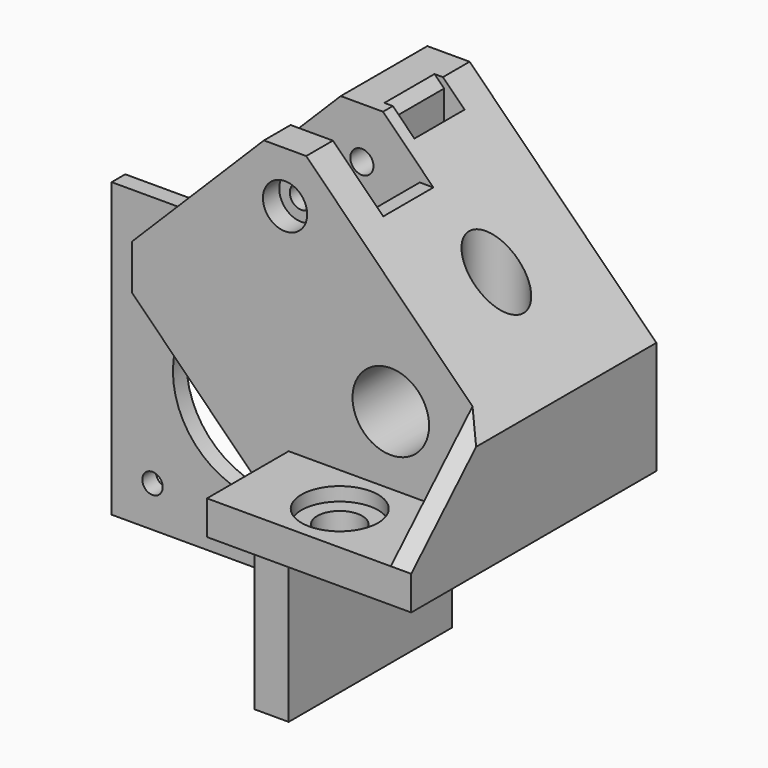
from build123d import *

# Parameters (mm, degrees)
F5_DEPTH        = 30
F7_DEPTH        = 27.5
F9_DEPTH        = 9.2
F11_DEPTH       = 9.2
F13_D           = 6.6
F13_CBORE_D     = 11.25
F13_CBORE_DEPTH = 27
F15_R           = 4
F16_DEPTH       = 39.001
F18_D           = 6.6
F18_CBORE_D     = 11.25
F18_CBORE_DEPTH = 2
F20_DEPTH       = 15
F22_D           = 6.6
F22_CBORE_D     = 11.25
F22_CBORE_DEPTH = 2
F24_DEPTH       = 3.001
F25_R           = 1.5
F25_R_2         = 12.5
F26_DEPTH       = 45.001
F28_D           = 3.4
F28_DEPTH       = 20
F28_CBORE_D     = 6.5
F28_CBORE_DEPTH = 3
F28_TIP         = 1.0214630523
F30_D           = 3.4
F30_DEPTH       = 20
F30_CBORE_D     = 6.5
F30_CBORE_DEPTH = 3
F30_TIP         = 1.0214630523
F31_SIZE        = 5


# Not quite as in the source:
# - a feature of the source that left no trace in its solid (it failed there, or was rolled back) is left out


with BuildPart() as f5:
    # F4 (on Front) → F5 (new body)
    with BuildSketch(Plane.XZ):
        Polygon((35, 46.5766017178), (7.5766017178, 74), (1.3633982822, 74), (-18.03, 54.6066017178), (-18.03, 43), (-43, 43), (-43, 0), (5, 0), (5, 30), (35, 30), align=None)
    extrude(amount=F5_DEPTH)

    # F6 (on face) → F7 (cut)
    with BuildSketch(Plane.XZ.offset(30)):
        Polygon((-43, 43), (-43, 0), (0, 0), (0, 30), (-18.03, 48.03), (-18.03, 43), align=None)
    extrude(amount=-F7_DEPTH, mode=Mode.SUBTRACT)

    # F8 (on offset) → F9 (cut)
    with BuildSketch(Plane.XZ.offset(14.1)):
        with BuildLine():
            Line((-18.03, 48.03), (-2.7734474577, 32.7734474577))
            Line((-2.7734474577, 32.7734474577), (9.5961081783, 47.0624990203))
            ThreePointArc((9.5961081783, 47.0624990203), (11.1595399436, 50.3961633531), (10.75, 54.0553864678))
            Line((10.75, 54.0553864678), (10.75, 70.8266017178))
            Line((10.75, 70.8266017178), (7.5766017178, 74))
            Line((7.5766017178, 74), (6.3357864376, 74))
            Line((6.3357864376, 74), (7.75, 72.5857864376))
            Line((7.75, 72.5857864376), (7.75, 61.4142135624))
            Line((7.75, 61.4142135624), (6.3357864376, 60))
            Line((6.3357864376, 60), (1.5055339059, 60))
            Line((1.5055339059, 60), (-5.5655339059, 67.0710678119))
            Line((-5.5655339059, 67.0710678119), (-18.03, 54.6066017178))
            Line((-18.03, 54.6066017178), (-18.03, 48.03))
        make_face()
    extrude(amount=-F9_DEPTH, mode=Mode.SUBTRACT)

    # F10 (on offset) → F11 (cut)
    with BuildSketch(Plane.XZ.offset(15.9)):
        with BuildLine():
            Line((1.3633982822, 74), (-16.6157864376, 56.0208152802))
            Line((-16.6157864376, 56.0208152802), (5.2500150699, 58.035865284))
            ThreePointArc((5.2500150699, 58.035865284), (10.7501324864, 60.7720041941), (12.97, 66.5))
            Line((12.97, 66.5), (12.97, 66.6066017178))
            Line((12.97, 66.6066017178), (14.97, 66.6066017178))
            Line((14.97, 66.6066017178), (7.5766017178, 74))
            Line((7.5766017178, 74), (1.3633982822, 74))
        make_face()
    extrude(amount=F11_DEPTH, mode=Mode.SUBTRACT)

    # F13 (through all)
    with Locations(Plane.XZ.offset(30)):
        with Locations((20, 45)):
            CounterBoreHole(F13_D / 2, F13_CBORE_D / 2, F13_CBORE_DEPTH)

    # F15 (on offset) → F16 (cut, through all)
    with BuildSketch(Plane(origin=(0, 0, 35), x_dir=(1, 0, 0), z_dir=(0, 0, -1))):
        with Locations((23.5, 15)):
            Circle(F15_R)
    extrude(amount=-F16_DEPTH, mode=Mode.SUBTRACT)

    # F18 (through all)
    with Locations(Plane(origin=(0, 0, 0), x_dir=(0, -1, 0), z_dir=(-1, 0, 0))):
        with Locations((16.25, 15)):
            CounterBoreHole(F18_D / 2, F18_CBORE_D / 2, F18_CBORE_DEPTH)

    # F19 (on face) → F20 (join)
    with BuildSketch(Plane.XZ.offset(30)):
        Polygon((5, 30), (35, 30), (35, 35), (35, 46.5766017178), (32, 49.5766017178), (32, 35), (5, 35), align=None)
    extrude(amount=F20_DEPTH)

    # F22 (through all)
    with Locations(Plane.XY.offset(35)):
        with Locations((18.5, -37.5)):
            CounterBoreHole(F22_D / 2, F22_CBORE_D / 2, F22_CBORE_DEPTH)

    # F23 (on face) → F24 (cut, through all)
    with BuildSketch(Plane(origin=(32, 0, 0), x_dir=(0, -1, 0), z_dir=(-1, 0, 0))):
        Polygon((45, 49.5766017178), (30, 49.5766017178), (45, 35), align=None)
    extrude(amount=-F24_DEPTH, mode=Mode.SUBTRACT)

    # F25 (on face) → F26 (cut, through all)
    with BuildSketch(Plane(origin=(0, 0, 0), x_dir=(-1, 0, 0), z_dir=(0, 1, 0))):
        with Locations((37, 37)):
            Circle(F25_R)
        with Locations((37, 6)):
            Circle(F25_R)
        with Locations((6, 6)):
            Circle(F25_R)
        with Locations((21.5, 21.5)):
            Circle(F25_R_2)
    extrude(amount=-F26_DEPTH, mode=Mode.SUBTRACT)

    # F28
    with Locations(Plane.XZ.offset(30)):
        with Locations((4.47, 66.5)):
            CounterBoreHole(F28_D / 2, F28_CBORE_D / 2, F28_CBORE_DEPTH, depth=F28_DEPTH)
            with Locations((0, 0, -(F28_DEPTH + F28_TIP / 2))):  # 118° drill point
                Cone(0, F28_D / 2, F28_TIP, mode=Mode.SUBTRACT)

    # F30
    with Locations(Plane(origin=(0, 0, 0), x_dir=(-1, 0, 0), z_dir=(0, 1, 0))):
        with Locations((-4.47, 51.5), (10.53, 51.5)):
            CounterBoreHole(F30_D / 2, F30_CBORE_D / 2, F30_CBORE_DEPTH, depth=F30_DEPTH)
            with Locations((0, 0, -(F30_DEPTH + F30_TIP / 2))):  # 118° drill point
                Cone(0, F30_D / 2, F30_TIP, mode=Mode.SUBTRACT)

    # F31
    f31_edges = [f5.edges().sort_by_distance(p)[0] for p in [
        (-18.03, -1.25, 43),
    ]]
    chamfer(f31_edges, length=F31_SIZE)


solid = f5.part
